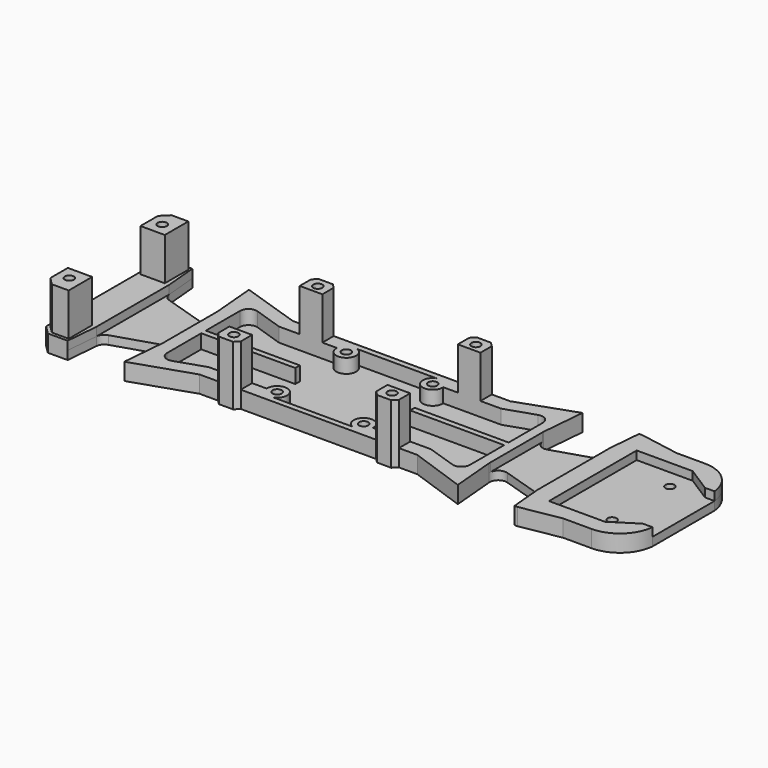
from build123d import *

# Parameters (mm, degrees)
F0_R      = 1.6
F1_DEPTH  = 3
F2_R      = 1.6
F3_DEPTH  = 3
F5_DEPTH  = 5
F6_R      = 1.6
F7_DEPTH  = 15
F8_R      = 1.6
F9_DEPTH  = 15
F10_R     = 1.6
F11_DEPTH = 3


# Not quite as in the source:
# - ends of sketch curves that miss each other by under 0.0002 mm in the source are joined


with BuildPart() as f1:
    # F0 (on Top) → F1 (new body)
    with BuildSketch(Plane.XY):
        with BuildLine():
            Line((14.627107, -22), (17.127107, -22))
            Line((17.127107, -22), (18.627107, -20.5))
            Line((18.627107, -20.5), (25.127107, -20.5))
            Line((25.127107, -20.5), (45.0241078911, -27.4989450371))
            Line((45.0241078911, -27.4989450371), (43.6660160882, -11.9758846978))
            ThreePointArc((43.6660160882, -11.9758846978), (44.7775912608, -9.3741530598), (47.5585796034, -8.853854377))
            Line((47.5585796034, -8.853854377), (61.9330823218, -13.3964056938))
            ThreePointArc((61.9330823218, -13.3964056938), (63.3693673107, -14.3799598647), (64.0176869952, -15.9955015581))
            Line((64.0176869952, -15.9955015581), (65.0242001884, -27.5))
            Line((65.0242001884, -27.5), (66.027107, -27.5))
            Line((66.027107, -27.5), (80.230626, -25))
            Line((80.230626, -25), (90.230626, -25))
            ThreePointArc((90.230626, -25), (98.634494133, -21.7533777834), (102.6728926683, -13.7000000645))
            Line((102.6728926683, -13.7000000645), (102.672892, 13.7))
            ThreePointArc((102.672892, 13.7), (98.634494133, 21.7533777834), (90.230626, 25))
            Line((90.230626, 25), (80.230626, 25))
            Line((80.230626, 25), (66.027107, 27.5))
            Line((66.027107, 27.5), (65.0242001884, 27.5))
            Line((65.0242001884, 27.5), (64.0176869952, 15.9955015581))
            ThreePointArc((64.0176869952, 15.9955015581), (63.3693673107, 14.3799598647), (61.9330823218, 13.3964056938))
            Line((61.9330823218, 13.3964056938), (47.5585796034, 8.853854377))
            ThreePointArc((47.5585796034, 8.853854377), (44.7775912608, 9.3741530598), (43.6660160882, 11.9758846978))
            Line((43.6660160882, 11.9758846978), (45.0241078911, 27.4989450371))
            Line((45.0241078911, 27.4989450371), (25.127107, 20.5))
            Line((25.127107, 20.5), (18.627107, 20.5))
            Line((18.627107, 20.5), (17.127107, 22))
            Line((17.127107, 22), (14.627107, 22))
            Line((14.627107, 22), (12.127107, 22))
            Line((12.127107, 22), (10.627107, 20.5))
            Line((10.627107, 20.5), (-37.172893, 20.5))
            Line((-37.172893, 20.5), (-38.672893, 22))
            Line((-38.672893, 22), (-43.672893, 22))
            Line((-43.672893, 22), (-45.172893, 20.5))
            Line((-45.172893, 20.5), (-51.672893, 20.5))
            Line((-51.672893, 20.5), (-72.672893, 27.5))
            Line((-72.672893, 27.5), (-71.3147088998, 11.9758846978))
            ThreePointArc((-71.3147088998, 11.9758846978), (-72.4262840724, 9.3741530598), (-75.207272415, 8.853854377))
            Line((-75.207272415, 8.853854377), (-89.5817751334, 13.3964056938))
            ThreePointArc((-89.5817751334, 13.3964056938), (-91.0180601223, 14.3799598647), (-91.6663798068, 15.9955015581))
            Line((-91.6663798068, 15.9955015581), (-92.672893, 27.5))
            Line((-92.672893, 27.5), (-99.672893, 27.5))
            Line((-99.672893, 27.5), (-102.672893, 24.5))
            Line((-102.672893, 24.5), (-102.672893, -24.5))
            Line((-102.672893, -24.5), (-99.672893, -27.5))
            Line((-99.672893, -27.5), (-92.672893, -27.5))
            Line((-92.672893, -27.5), (-91.6663798068, -15.9955015581))
            ThreePointArc((-91.6663798068, -15.9955015581), (-91.0180601223, -14.3799598647), (-89.5817751334, -13.3964056938))
            Line((-89.5817751334, -13.3964056938), (-75.207272415, -8.853854377))
            ThreePointArc((-75.207272415, -8.853854377), (-72.4262840724, -9.3741530598), (-71.3147088998, -11.9758846978))
            Line((-71.3147088998, -11.9758846978), (-72.672893, -27.5))
            Line((-72.672893, -27.5), (-51.672893, -20.5))
            Line((-51.672893, -20.5), (-45.172893, -20.5))
            Line((-45.172893, -20.5), (-43.672893, -22))
            Line((-43.672893, -22), (-41.172893, -22))
            Line((-41.172893, -22), (-38.672893, -22))
            Line((-38.672893, -22), (-37.172893, -20.5))
            Line((-37.172893, -20.5), (10.627107, -20.5))
            Line((10.627107, -20.5), (12.127107, -22))
            Line((12.127107, -22), (14.627107, -22))
        make_face()
        with Locations((-97.672893, -20.5)):
            Circle(F0_R, mode=Mode.SUBTRACT)
        with Locations((-41.172893, -18.5)):
            Circle(F0_R, mode=Mode.SUBTRACT)
        with Locations((-28.522893, -15.25)):
            Circle(F0_R, mode=Mode.SUBTRACT)
        with Locations((14.627107, -18.5)):
            Circle(F0_R, mode=Mode.SUBTRACT)
        with Locations((1.977107, -15.25)):
            Circle(F0_R, mode=Mode.SUBTRACT)
        with Locations((87.672892, -12.75)):
            Circle(F0_R, mode=Mode.SUBTRACT)
        with Locations((-97.672893, 20.5)):
            Circle(F0_R, mode=Mode.SUBTRACT)
        with Locations((-28.522893, 15.25)):
            Circle(F0_R, mode=Mode.SUBTRACT)
        with Locations((-41.172893, 18.5)):
            Circle(F0_R, mode=Mode.SUBTRACT)
        with Locations((87.672892, 12.75)):
            Circle(F0_R, mode=Mode.SUBTRACT)
        with Locations((1.977107, 15.25)):
            Circle(F0_R, mode=Mode.SUBTRACT)
        with Locations((14.627107, 18.5)):
            Circle(F0_R, mode=Mode.SUBTRACT)
    extrude(amount=F1_DEPTH)

    # F2 (on face) → F3 (join)
    with BuildSketch(Plane.XY.offset(3)):
        Polygon((-91.672392004, -16.0642212863), (-91.672392004, 16.0642212863), (-92.672893, 27.5), (-99.672893, 27.5), (-102.672893, 24.5), (-102.672893, -24.5), (-99.672893, -27.5), (-92.672893, -27.5), align=None)
        with Locations((-97.672893, -20.5)):
            Circle(F2_R, mode=Mode.SUBTRACT)
        with Locations((-97.672893, 20.5)):
            Circle(F2_R, mode=Mode.SUBTRACT)
        with BuildLine():
            ThreePointArc((-71.3147088998, 11.9758846978), (-71.3032929941, 11.7144174696), (-71.3147088998, 11.4529502413))
            Line((-71.3147088998, 11.4529502413), (-71.3147088998, -11.4529502413))
            ThreePointArc((-71.3147088998, -11.4529502413), (-71.3032929941, -11.7144174696), (-71.3147088998, -11.9758846978))
            Line((-71.3147088998, -11.9758846978), (-72.672893, -27.5))
            Line((-72.672893, -27.5), (-51.672893, -20.5))
            Line((-51.672893, -20.5), (-45.172893, -20.5))
            Line((-45.172893, -20.5), (-43.672893, -22))
            Line((-43.672893, -22), (-38.672893, -22))
            Line((-38.672893, -22), (-37.172893, -20.5))
            Line((-37.172893, -20.5), (10.627107, -20.5))
            Line((10.627107, -20.5), (12.127107, -22))
            Line((12.127107, -22), (17.127107, -22))
            Line((17.127107, -22), (18.627107, -20.5))
            Line((18.627107, -20.5), (25.127107, -20.5))
            Line((25.127107, -20.5), (45.0241078911, -27.4989450371))
            Line((45.0241078911, -27.4989450371), (43.6660160882, -11.9758846978))
            ThreePointArc((43.6660160882, -11.9758846978), (43.6546001825, -11.7144174696), (43.6660160882, -11.4529502413))
            Line((43.6660160882, -11.4529502413), (43.6660160882, 11.4529502413))
            ThreePointArc((43.6660160882, 11.4529502413), (43.6546001825, 11.7144174696), (43.6660160882, 11.9758846978))
            Line((43.6660160882, 11.9758846978), (45.0241078911, 27.4989450371))
            Line((45.0241078911, 27.4989450371), (25.127107, 20.5))
            Line((25.127107, 20.5), (18.627107, 20.5))
            Line((18.627107, 20.5), (17.127107, 22))
            Line((17.127107, 22), (12.127107, 22))
            Line((12.127107, 22), (10.627107, 20.5))
            Line((10.627107, 20.5), (-37.172893, 20.5))
            Line((-37.172893, 20.5), (-38.672893, 22))
            Line((-38.672893, 22), (-43.672893, 22))
            Line((-43.672893, 22), (-45.172893, 20.5))
            Line((-45.172893, 20.5), (-51.672893, 20.5))
            Line((-51.672893, 20.5), (-72.672893, 27.5))
            Line((-72.672893, 27.5), (-71.3147088998, 11.9758846978))
        make_face()
        with Locations((-41.172893, -18.5)):
            Circle(F2_R, mode=Mode.SUBTRACT)
        with Locations((-28.522893, -15.25)):
            Circle(F2_R, mode=Mode.SUBTRACT)
        with Locations((14.627107, -18.5)):
            Circle(F2_R, mode=Mode.SUBTRACT)
        with Locations((1.977107, -15.25)):
            Circle(F2_R, mode=Mode.SUBTRACT)
        with Locations((-28.522893, 15.25)):
            Circle(F2_R, mode=Mode.SUBTRACT)
        with Locations((-41.172893, 18.5)):
            Circle(F2_R, mode=Mode.SUBTRACT)
        with Locations((1.977107, 15.25)):
            Circle(F2_R, mode=Mode.SUBTRACT)
        with Locations((14.627107, 18.5)):
            Circle(F2_R, mode=Mode.SUBTRACT)
        with BuildLine():
            Line((65.0242001884, 27.5), (64.0236991924, 16.0642212863))
            Line((64.0236991924, 16.0642212863), (64.0236991924, -16.0642212863))
            Line((64.0236991924, -16.0642212863), (65.0242001884, -27.5))
            Line((65.0242001884, -27.5), (66.027107, -27.5))
            Line((66.027107, -27.5), (80.230626, -25))
            Line((80.230626, -25), (90.230626, -25))
            ThreePointArc((90.230626, -25), (98.634494133, -21.7533777834), (102.6728926683, -13.7000000645))
            Line((102.6728926683, -13.7000000645), (102.672892, 13.7))
            ThreePointArc((102.672892, 13.7), (98.634494037, 21.7533778706), (90.230626, 25))
            Line((90.230626, 25), (80.230626, 25))
            Line((80.230626, 25), (66.027107, 27.5))
            Line((66.027107, 27.5), (65.0242001884, 27.5))
        make_face()
        with Locations((87.672892, -12.75)):
            Circle(F2_R, mode=Mode.SUBTRACT)
        with Locations((87.672892, 12.75)):
            Circle(F2_R, mode=Mode.SUBTRACT)
    extrude(amount=F3_DEPTH)

    # F4 (on face) → F5 (cut)
    with BuildSketch(Plane.XY.offset(6)):
        with BuildLine():
            Line((-52.4842813008, 15.5), (-62.7658474735, 18.9271887242))
            ThreePointArc((-62.7658474735, 18.9271887242), (-65.4686616256, 18.5148653856), (-66.7145307716, 16.0811388301))
            Line((-66.7145307716, 16.0811388301), (-66.7145307716, 1))
            Line((-66.7145307716, 1), (-33.522893, 1))
            Line((-33.522893, 1), (-33.522893, -1))
            Line((-33.522893, -1), (-66.7145307716, -1))
            Line((-66.7145307716, -1), (-66.7145307716, -16.0811388301))
            ThreePointArc((-66.7145307716, -16.0811388301), (-65.4686616256, -18.5148653856), (-62.7658474735, -18.9271887242))
            Line((-62.7658474735, -18.9271887242), (-52.4842813008, -15.5))
            Line((-52.4842813008, -15.5), (-32.0139530109, -15.5))
            ThreePointArc((-32.0139530109, -15.5), (-26.6651416689, -12.2837296159), (-27.2238548943, -18.5))
            Line((-27.2238548943, -18.5), (0.6780688943, -18.5))
            ThreePointArc((0.6780688943, -18.5), (0.1193556689, -12.2837296159), (5.4681670109, -15.5))
            Line((5.4681670109, -15.5), (25.9384953008, -15.5))
            Line((25.9384953008, -15.5), (36.2200614735, -18.9271887242))
            ThreePointArc((36.2200614735, -18.9271887242), (38.9228756256, -18.5148653856), (40.1687447716, -16.0811388301))
            Line((40.1687447716, -16.0811388301), (40.1687447716, -1))
            Line((40.1687447716, -1), (6.977107, -1))
            Line((6.977107, -1), (6.977107, 1))
            Line((6.977107, 1), (40.1687447716, 1))
            Line((40.1687447716, 1), (40.1687447716, 16.0811388301))
            ThreePointArc((40.1687447716, 16.0811388301), (38.9228756256, 18.5148653856), (36.2200614735, 18.9271887242))
            Line((36.2200614735, 18.9271887242), (25.9384953008, 15.5))
            Line((25.9384953008, 15.5), (5.4681670109, 15.5))
            ThreePointArc((5.4681670109, 15.5), (0.1193556689, 12.2837296159), (0.6780688943, 18.5))
            Line((0.6780688943, 18.5), (-27.2238548943, 18.5))
            ThreePointArc((-27.2238548943, 18.5), (-26.6651416689, 12.2837296159), (-32.0139530109, 15.5))
            Line((-32.0139530109, 15.5), (-52.4842813008, 15.5))
        make_face()
    extrude(amount=-F5_DEPTH, mode=Mode.SUBTRACT)

    # F6 (on face) → F7 (join)
    with BuildSketch(Plane.XY.offset(6)):
        Polygon((-101.7832774669, 16.0122346133), (-93.1889638305, 16.0122346133), (-93.1889638305, 26.3799782842), (-99.1367772222, 26.3799782842), (-101.7832774669, 23.7334780395), align=None)
        with Locations((-97.672893, 20.5)):
            Circle(F6_R, mode=Mode.SUBTRACT)
        Polygon((-99.1367772222, -26.3799782842), (-93.1889638305, -26.3799782842), (-93.1889638305, -16.0122346133), (-101.7832774669, -16.0122346133), (-101.7832774669, -23.7334780395), align=None)
        with Locations((-97.672893, -20.5)):
            Circle(F6_R, mode=Mode.SUBTRACT)
    extrude(amount=F7_DEPTH)

    # F8 (on face) → F9 (join)
    with BuildSketch(Plane.XY.offset(6)):
        Polygon((-43.672893, 22), (-45.172893, 20.5), (-45.172893, 15.5), (-37.172893, 15.5), (-37.172893, 20.5), (-38.672893, 22), align=None)
        with Locations((-41.172893, 18.5)):
            Circle(F8_R, mode=Mode.SUBTRACT)
        Polygon((18.627107, 15.5), (18.627107, 20.5), (17.127107, 22), (12.127107, 22), (10.627107, 20.5), (10.627107, 15.5), align=None)
        with Locations((14.627107, 18.5)):
            Circle(F8_R, mode=Mode.SUBTRACT)
        Polygon((10.627107, -15.5), (10.627107, -20.5), (12.127107, -22), (17.127107, -22), (18.627107, -20.5), (18.627107, -15.5), align=None)
        with Locations((14.627107, -18.5)):
            Circle(F8_R, mode=Mode.SUBTRACT)
        Polygon((-38.672893, -22), (-37.172893, -20.5), (-37.172893, -15.5), (-45.172893, -15.5), (-45.172893, -20.5), (-43.672893, -22), align=None)
        with Locations((-41.172893, -18.5)):
            Circle(F8_R, mode=Mode.SUBTRACT)
    extrude(amount=F9_DEPTH)

    # F10 (on face) → F11 (cut)
    with BuildSketch(Plane.XY.offset(6)):
        Polygon((99.2892167695, -13.7000000645), (102.6728926683, -13.7000000645), (102.672892, 13.7), (99.2892167695, 13.7000000645), (90.4360420234, 19.3481259693), (70.672892, 19.3481259693), (70.672892, -19.3481259693), (90.4360420234, -19.3481259693), align=None)
        with Locations((87.672892, -12.75)):
            Circle(F10_R, mode=Mode.SUBTRACT)
        with Locations((87.672892, 12.75)):
            Circle(F10_R, mode=Mode.SUBTRACT)
    extrude(amount=-F11_DEPTH, mode=Mode.SUBTRACT)


solid = f1.part
